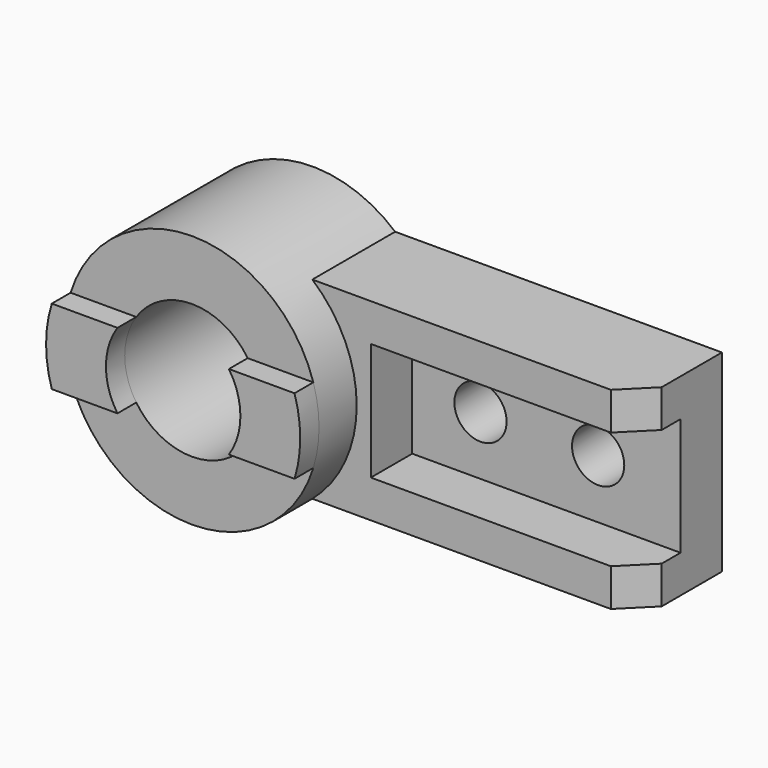
from build123d import *
from build123d import SkipClean  # not in build123d's __all__

# Parameters (mm, degrees)
F0_R          = 54
F0_R_2        = 28.575
F1_DEPTH      = 32
F3_DEPTH      = 10
F5_DEPTH      = 32
F5_DEPTH_BACK = 12
F4_W          = 114
F4_H          = 50
F4_R          = 11.1
F6_DEPTH      = 32
F7_DEPTH      = 10
F9_DEPTH      = 95.001


# Not quite as in the source:
# - after a boolean that leaves OpenCascade's solid faulty, fix() repairs it


with BuildPart() as f1:
    # F0 (on Front) → F1 (new body, symmetric)
    with BuildSketch(Plane.XZ):
        Circle(F0_R)
        Circle(F0_R_2, mode=Mode.SUBTRACT)
    extrude(amount=F1_DEPTH, both=True)

    # F2 (on face) → F3 (join)
    with BuildSketch(Plane.XZ.offset(32)):
        with BuildLine():
            ThreePointArc((-51.575188, 16), (-54, 0), (-51.575188, -16))
            Line((-51.575188, -16), (-23.675528, -16))
            ThreePointArc((-23.675528, -16), (-28.575, 0), (-23.675528, 16))
            Line((-23.675528, 16), (-51.575188, 16))
        make_face()
        with BuildLine():
            ThreePointArc((23.675528, 16), (28.575, 0), (23.675528, -16))
            Line((23.675528, -16), (51.575188, -16))
            ThreePointArc((51.575188, -16), (54, 0), (51.575188, 16))
            Line((51.575188, 16), (23.675528, 16))
        make_face()
    with SkipClean():  # cleaning this boolean's faces spoils the solid; the shape is the same uncleaned
        extrude(amount=F3_DEPTH)

    # F4 (on Front) → F5 (join, two sides)
    with BuildSketch(Plane.XZ) as f5_sk:
        with BuildLine():
            Line((174, 41), (35.142567, 41))
            ThreePointArc((35.142567, 41), (54, 0), (35.142567, -41))
            Line((35.142567, -41), (174, -41))
            Line((174, -41), (174, -25))
            Line((174, -25), (60, -25))
            Line((60, -25), (60, 25))
            Line((60, 25), (174, 25))
            Line((174, 25), (174, 41))
        make_face()
    extrude(amount=-F5_DEPTH)
    extrude(f5_sk.sketch, amount=F5_DEPTH_BACK)

    add(f1.part.fix(), mode=Mode.REPLACE)

    # F4 (on Front) → F6 (join)
    with BuildSketch(Plane.XZ):
        with Locations((117, 0)):
            Rectangle(F4_W, F4_H)
        with Locations((89, 0)):
            Circle(F4_R, mode=Mode.SUBTRACT)
        with Locations((139, 0)):
            Circle(F4_R, mode=Mode.SUBTRACT)
    extrude(amount=-F6_DEPTH)

    # F4 (on Front) → F7 (cut)
    with BuildSketch(Plane.XZ):
        with Locations((117, 0)):
            Rectangle(F4_W, F4_H)
        with Locations((89, 0)):
            Circle(F4_R, mode=Mode.SUBTRACT)
        with Locations((139, 0)):
            Circle(F4_R, mode=Mode.SUBTRACT)
    extrude(amount=-F7_DEPTH, mode=Mode.SUBTRACT)

    # F8 (on face) → F9 (cut, through all)
    with BuildSketch(Plane(origin=(0, 0, -41), x_dir=(1, 0, 0), z_dir=(0, 0, -1))):
        Polygon((174, 12), (162, 12), (174, 0), align=None)
    extrude(amount=-F9_DEPTH, mode=Mode.SUBTRACT)


solid = f1.part
